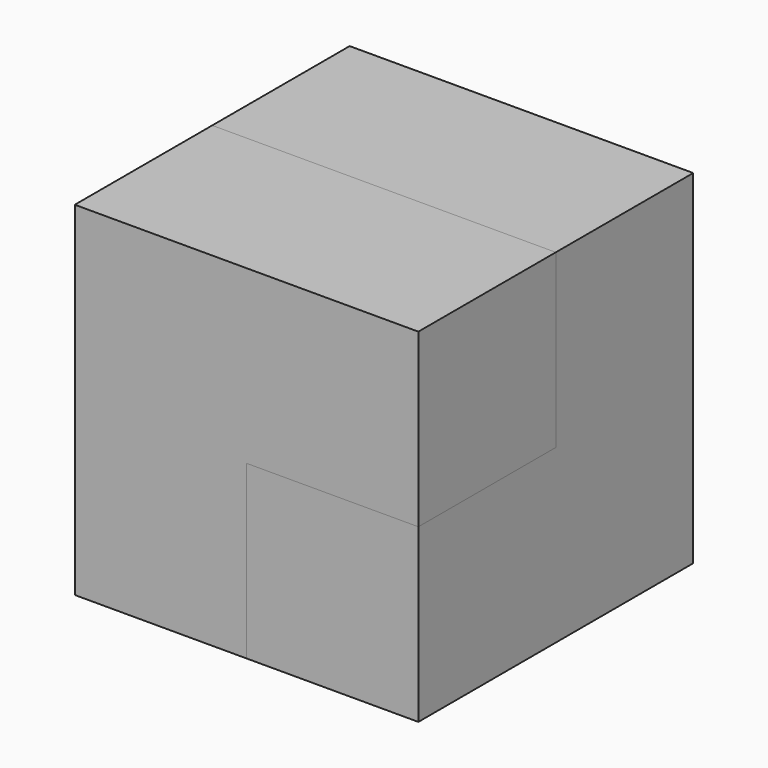
from build123d import *

# Parameters (mm, degrees)
F2_DEPTH      = 10.16
F3_W          = 10.16
F3_H          = 10.16
F4_DEPTH      = 10.16
F5_W          = 20.32
F5_H          = 20.32
F6_DEPTH      = 10.16
F6_DEPTH_BACK = 10.16


# Not quite as in the source:
# - a variable given as a bare number and used for a length is read in inches; the dataset says mm whatever the document's units were


with BuildPart() as f2:
    # F1 (on Right) → F2 (new body)
    with BuildSketch(Plane.YZ):
        Polygon((10.16, 0), (0, 0), (0, 10.16), (-10.16, 10.16), (-10.16, -10.16), (10.16, -10.16), align=None)
    extrude(amount=-F2_DEPTH)

    # F3 (on face) → F4 (join)
    with BuildSketch(Plane.YZ):
        with Locations((-5.08, 5.08)):
            Rectangle(F3_W, F3_H)
    extrude(amount=F4_DEPTH)


with BuildPart() as f6:
    # F5 (on Top) → F6 (new body, two sides)
    with BuildSketch(Plane.XY) as f6_sk:
        Rectangle(F5_W, F5_H)
    extrude(amount=F6_DEPTH)
    extrude(f6_sk.sketch, amount=-F6_DEPTH_BACK)

    # F7: cut F2
    add(f2.part, mode=Mode.SUBTRACT)


solid = Compound([f2.part, f6.part])
